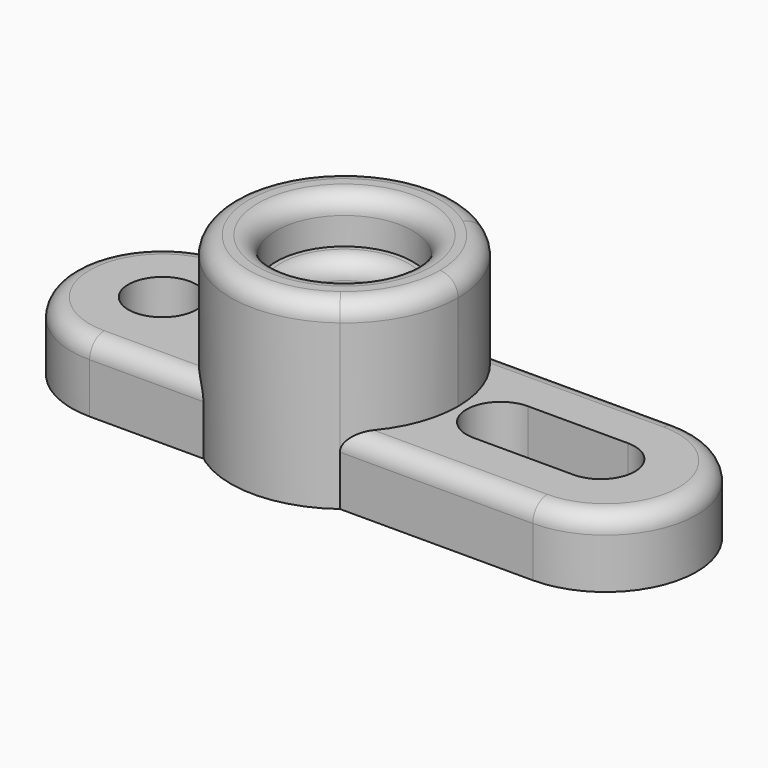
from build123d import *

# Parameters (mm, degrees)
F0_R     = 9.525
F1_DEPTH = 19.05
F0_R_2   = 19.05
F2_DEPTH = 50.8
F0_R_3   = 12.7
F3_DEPTH = 38.1
F4_R     = 5.08
F4_2_R   = 5.08
F4_3_R   = 5.08


# Not quite as in the source:
# - a feature names something its author has since deleted; it is built from what else it names


with BuildPart() as f1:
    # F0 (on Top) → F1 (new body)
    with BuildSketch(Plane.XY):
        with BuildLine():
            ThreePointArc((-19.05, -25.4), (-31.75, 0), (-19.05, 25.4))
            Line((-19.05, 25.4), (-50.8, 25.4))
            ThreePointArc((-50.8, 25.4), (-76.2, 0), (-50.8, -25.4))
            Line((-50.8, -25.4), (-19.05, -25.4))
        make_face()
        with Locations((-50.8, 0)):
            Circle(F0_R, mode=Mode.SUBTRACT)
    extrude(amount=F1_DEPTH)

    # F4
    f4_edges = [f1.edges().sort_by_distance(p)[0] for p in [
        (-76.2, 0, 19.05),
    ]]
    fillet(f4_edges, radius=F4_R)


with BuildPart() as f1b:
    # F0 (on Top) → F1, piece 2 (new body)
    with BuildSketch(Plane.XY):
        with BuildLine():
            ThreePointArc((19.05, 25.4), (28.3980633142, 14.1990316571), (31.75, 0))
            ThreePointArc((31.75, 0), (28.3980633142, -14.1990316571), (19.05, -25.4))
            Line((19.05, -25.4), (72.898, -25.4))
            ThreePointArc((72.898, -25.4), (98.298, 0), (72.898, 25.4))
            Line((72.898, 25.4), (19.05, 25.4))
        make_face()
        with BuildLine():
            ThreePointArc((43.6129720223, -9.525), (34.0879720223, 0), (43.6129720223, 9.525))
            Line((43.6129720223, 9.525), (71.5529720223, 9.525))
            ThreePointArc((71.5529720223, 9.525), (81.0779720223, 0), (71.5529720223, -9.525))
            Line((71.5529720223, -9.525), (43.6129720223, -9.525))
        make_face(mode=Mode.SUBTRACT)
    extrude(amount=F1_DEPTH)

    # F4#2
    f4_2_edges = [f1b.edges().sort_by_distance(p)[0] for p in [
        (98.298, 0, 19.05),
    ]]
    fillet(f4_2_edges, radius=F4_2_R)


with BuildPart() as f2:
    # F0 (on Top) → F2 (new body)
    with BuildSketch(Plane.XY):
        with BuildLine():
            ThreePointArc((19.05, -25.4), (28.3980633142, -14.1990316571), (31.75, 0))
            ThreePointArc((31.75, 0), (28.3980633142, 14.1990316571), (19.05, 25.4))
            ThreePointArc((19.05, 25.4), (0, 31.75), (-19.05, 25.4))
            ThreePointArc((-19.05, 25.4), (-31.75, 0), (-19.05, -25.4))
            ThreePointArc((-19.05, -25.4), (0, -31.75), (19.05, -25.4))
        make_face()
        Circle(F0_R_2, mode=Mode.SUBTRACT)
    extrude(amount=F2_DEPTH)

    # F0 (on Top) → F3 (join)
    with BuildSketch(Plane.XY):
        Circle(F0_R_2)
        Circle(F0_R_3, mode=Mode.SUBTRACT)
    extrude(amount=F3_DEPTH)

    # F4#3
    f4_3_edges = [f2.edges().sort_by_distance(p)[0] for p in [
        (-19.05, -25.4, 50.8),
        (-19.05, 0, 50.8),
        (-12.7, 0, 38.1),
    ]]
    fillet(f4_3_edges, radius=F4_3_R)


solid = Compound([f1.part, f1b.part, f2.part])
